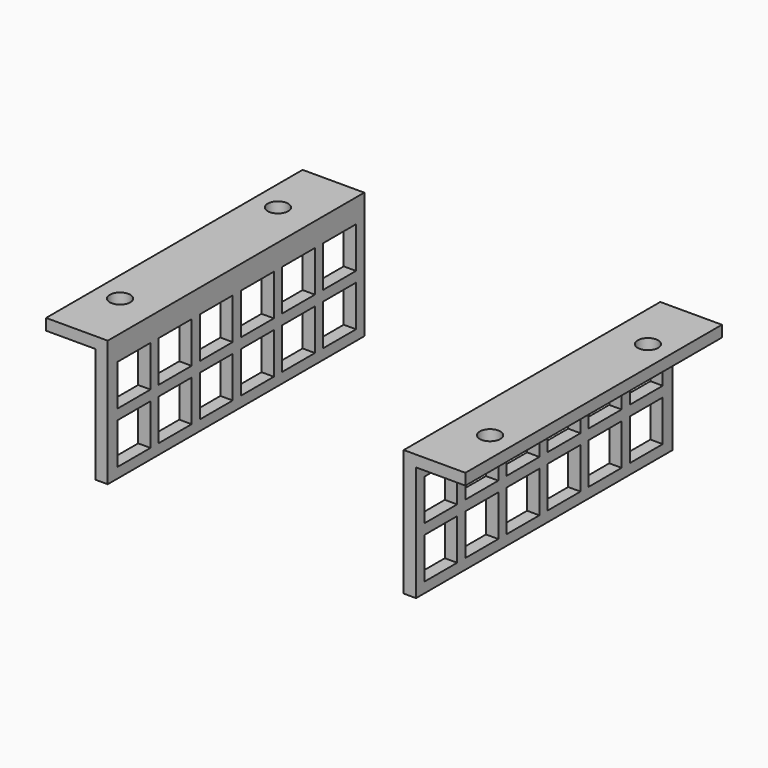
from build123d import *

# Parameters (mm, degrees)
F1_DEPTH = 39
F2_R     = 2.5
F3_DEPTH = 2.748386896
F4_W     = 10
F4_H     = 10
F5_DEPTH = 89.9998985683
F6_W     = 10
F6_H     = 10
F7_DEPTH = 89.9998985683


with BuildPart() as f1:
    # F0 (on Front) → F1 (new body, symmetric)
    with BuildSketch(Plane.XZ):
        Polygon((33.0240737289, -9.6249261405), (36.0251751605, -9.6249261405), (36.0251751605, 18.3750738595), (48.0240737289, 18.3750738595), (48.0240737289, 21.1234607555), (33.0240737289, 21.1234607555), align=None)
    extrude(amount=F1_DEPTH, both=True)


with BuildPart() as f1b:
    # F0 (on Front) → F1, piece 2 (new body, symmetric)
    with BuildSketch(Plane.XZ):
        Polygon((-53.9737234078, 21.1234607555), (-53.9737234078, 18.3750738595), (-41.9748248395, 18.3750738595), (-41.9748248395, -9.6249261405), (-38.9737234078, -9.6249261405), (-38.9737234078, 21.1234607555), align=None)
    extrude(amount=F1_DEPTH, both=True)


with BuildPart() as f3_tool:
    # F2 (on face) → F3 (new body, through all)
    with BuildSketch(Plane.XY.offset(21.1234607555)):
        with Locations((42.0246244447, -24)):
            Circle(F2_R)
        with Locations((42.0246244447, 24)):
            Circle(F2_R)
        with Locations((-47.9742741236, 24)):
            Circle(F2_R)
        with Locations((-47.9742741236, -24)):
            Circle(F2_R)
    extrude(amount=-F3_DEPTH)


with BuildPart() as f1_1:
    add(f1.part)

    # F3: cut by f3_tool
    add(f3_tool.part, mode=Mode.SUBTRACT)

    # F4 (on face) → F5 (cut, through all)
    with BuildSketch(Plane.YZ.offset(36.0251751605)):
        with Locations((-31.5, -2.1249261405)):
            Rectangle(F4_W, F4_H)
        with Locations((-31.5, 10.3750738595)):
            Rectangle(F4_W, F4_H)
        with Locations((-19, -2.1249261405)):
            Rectangle(F4_W, F4_H)
        with Locations((-19, 10.3750738595)):
            Rectangle(F4_W, F4_H)
        with Locations((-6.5, -2.1249261405)):
            Rectangle(F4_W, F4_H)
        with Locations((-6.5, 10.3750738595)):
            Rectangle(F4_W, F4_H)
        with Locations((6, -2.1249261405)):
            Rectangle(F4_W, F4_H)
        with Locations((6, 10.3750738595)):
            Rectangle(F4_W, F4_H)
        with Locations((18.5, -2.1249261405)):
            Rectangle(F4_W, F4_H)
        with Locations((18.5, 10.3750738595)):
            Rectangle(F4_W, F4_H)
        with Locations((31, -2.1249261405)):
            Rectangle(F4_W, F4_H)
        with Locations((31, 10.3750738595)):
            Rectangle(F4_W, F4_H)
    extrude(amount=-F5_DEPTH, mode=Mode.SUBTRACT)


with BuildPart() as f1b_1:
    add(f1b.part)

    # F3: cut by f3_tool
    add(f3_tool.part, mode=Mode.SUBTRACT)

    # F6 (on face) → F7 (cut, through all)
    with BuildSketch(Plane(origin=(-41.9748248395, 0, 0), x_dir=(0, -1, 0), z_dir=(-1, 0, 0))):
        with Locations((-31.5, -2.1249261405)):
            Rectangle(F6_W, F6_H)
        with Locations((-31.5, 10.3750738595)):
            Rectangle(F6_W, F6_H)
        with Locations((-19, -2.1249261405)):
            Rectangle(F6_W, F6_H)
        with Locations((-19, 10.3750738595)):
            Rectangle(F6_W, F6_H)
        with Locations((-6.5, -2.1249261405)):
            Rectangle(F6_W, F6_H)
        with Locations((-6.5, 10.3750738595)):
            Rectangle(F6_W, F6_H)
        with Locations((6, -2.1249261405)):
            Rectangle(F6_W, F6_H)
        with Locations((6, 10.3750738595)):
            Rectangle(F6_W, F6_H)
        with Locations((18.5, -2.1249261405)):
            Rectangle(F6_W, F6_H)
        with Locations((18.5, 10.3750738595)):
            Rectangle(F6_W, F6_H)
        with Locations((31, -2.1249261405)):
            Rectangle(F6_W, F6_H)
        with Locations((31, 10.3750738595)):
            Rectangle(F6_W, F6_H)
    extrude(amount=-F7_DEPTH, mode=Mode.SUBTRACT)


solid = Compound([f1_1.part, f1b_1.part])
